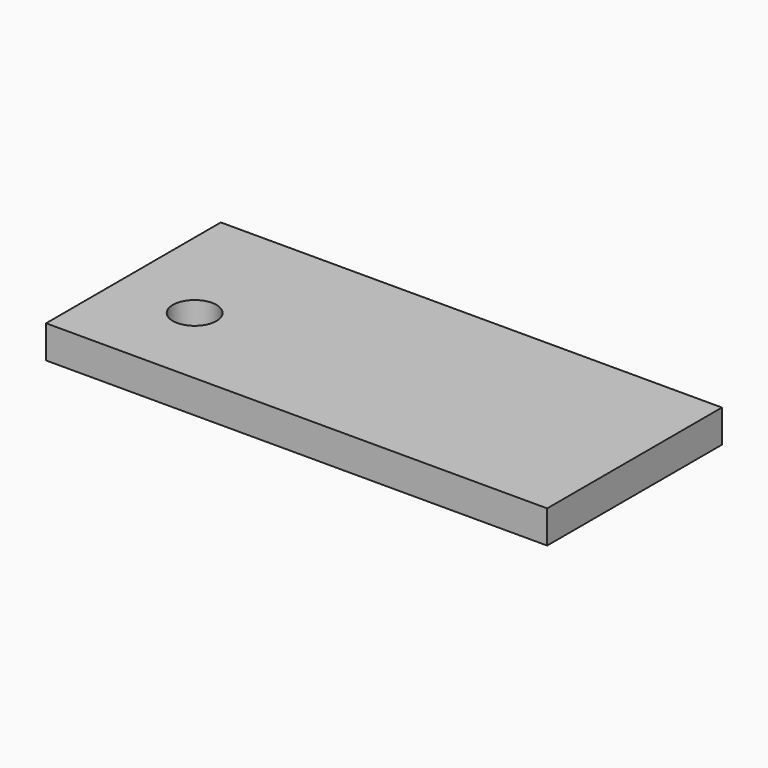
from build123d import *

# Parameters (mm, degrees)
F0_W          = 45.8885646038
F0_H          = 20
F1_DEPTH      = 3
F2_R          = 2
F3_DEPTH      = 52
F3_DEPTH_BACK = 25


# Not quite as in the source:
# - an extrude ends at something that could not be found from the text; its depth is read off the source's solid


with BuildPart() as f1:
    # F0 (on Top) → F1 (new body)
    with BuildSketch(Plane.XY):
        Rectangle(F0_W, F0_H)
    extrude(amount=F1_DEPTH)

    # F2 (on face) → F3 (cut, two sides)
    with BuildSketch(Plane.XY.offset(3)) as f3_sk:
        with Locations((-15.6491361558, -2.1147204097)):
            Circle(F2_R)
    extrude(amount=F3_DEPTH, mode=Mode.SUBTRACT)
    extrude(f3_sk.sketch, amount=-F3_DEPTH_BACK, mode=Mode.SUBTRACT)


solid = f1.part
